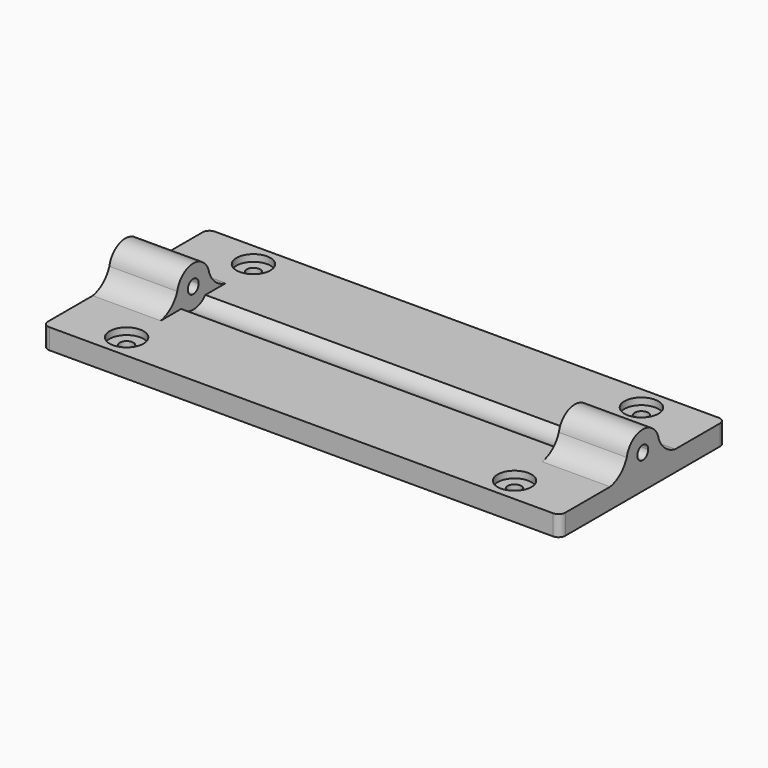
from build123d import *

# Parameters (mm, degrees)
F0_W          = 76.2
F0_H          = 30.48
F0_R          = 2.5
F2_DEPTH      = 3
F0_R_2        = 1
F3_DEPTH      = 2
F4_START      = 28.1
F4_DEPTH      = 10
F5_START      = -28.1
F5_DEPTH      = 10
F6_DEPTH      = 28.1
F6_DEPTH_BACK = 28.1
F7_R          = 1


with BuildPart() as f2:
    # F0 (on Top) → F2 (new body)
    with BuildSketch(Plane.XY):
        with Locations((0, 1.624652555)):
            Rectangle(F0_W, F0_H)
        with Locations((-28.57, -10.055347445)):
            Circle(F0_R, mode=Mode.SUBTRACT)
        with Locations((28.57, -10.055347445)):
            Circle(F0_R, mode=Mode.SUBTRACT)
        with Locations((-28.57, 13.304652555)):
            Circle(F0_R, mode=Mode.SUBTRACT)
        with Locations((28.57, 13.304652555)):
            Circle(F0_R, mode=Mode.SUBTRACT)
    extrude(amount=F2_DEPTH)

    # F0 (on Top) → F3 (join)
    with BuildSketch(Plane.XY):
        with Locations((28.57, 13.304652555)):
            Circle(F0_R)
        with Locations((28.57, 13.304652555)):
            Circle(F0_R_2, mode=Mode.SUBTRACT)
        with Locations((28.57, -10.055347445)):
            Circle(F0_R)
        with Locations((28.57, -10.055347445)):
            Circle(F0_R_2, mode=Mode.SUBTRACT)
        with Locations((-28.57, -10.055347445)):
            Circle(F0_R)
        with Locations((-28.57, -10.055347445)):
            Circle(F0_R_2, mode=Mode.SUBTRACT)
        with Locations((-28.57, 13.304652555)):
            Circle(F0_R)
        with Locations((-28.57, 13.304652555)):
            Circle(F0_R_2, mode=Mode.SUBTRACT)
    extrude(amount=F3_DEPTH)

    # F1 (on Right) → F4 (join)
    with BuildSketch(Plane.YZ.offset(F4_START)):
        with BuildLine():
            ThreePointArc((-1.3122499903, 5.5619300567), (-2.4969921778, 3.8736281168), (-4.365347445, 3))
            Line((-4.365347445, 3), (-0.6014154225, 3))
            ThreePointArc((-0.6014154225, 3), (-1.2561375211, 4.1979197446), (-1.3122499903, 5.5619300567))
        make_face()
        with BuildLine():
            Line((3.8707205325, 3), (7.634652555, 3))
            ThreePointArc((7.634652555, 3), (5.7662972877, 3.8736281168), (4.5815551003, 5.5619300567))
            ThreePointArc((4.5815551003, 5.5619300567), (4.6213486925, 5.2822165518), (4.634652555, 5))
            ThreePointArc((4.634652555, 5), (4.4371696319, 3.9295337307), (3.8707205325, 3))
        make_face()
        with BuildLine():
            ThreePointArc((-1.3122499903, 5.5619300567), (-1.2561375211, 4.1979197446), (-0.6014154225, 3))
            Line((-0.6014154225, 3), (3.8707205325, 3))
            ThreePointArc((3.8707205325, 3), (4.4371696319, 3.9295337307), (4.634652555, 5))
            ThreePointArc((4.634652555, 5), (4.6213486925, 5.2822165518), (4.5815551003, 5.5619300567))
            ThreePointArc((4.5815551003, 5.5619300567), (1.634652555, 8), (-1.3122499903, 5.5619300567))
        make_face()
        with BuildLine():
            ThreePointArc((1.634652555, 4), (0.9275457738, 5.7071067812), (2.634652555, 5))
            ThreePointArc((2.634652555, 5), (2.3417593362, 4.2928932188), (1.634652555, 4))
        make_face(mode=Mode.SUBTRACT)
    extrude(amount=F4_DEPTH)

    # F1 (on Right) → F5 (join)
    with BuildSketch(Plane.YZ.offset(F5_START)):
        with BuildLine():
            ThreePointArc((-1.3122499903, 5.5619300567), (-2.4969921778, 3.8736281168), (-4.365347445, 3))
            Line((-4.365347445, 3), (-0.6014154225, 3))
            ThreePointArc((-0.6014154225, 3), (-1.2561375211, 4.1979197446), (-1.3122499903, 5.5619300567))
        make_face()
        with BuildLine():
            Line((3.8707205325, 3), (7.634652555, 3))
            ThreePointArc((7.634652555, 3), (5.7662972877, 3.8736281168), (4.5815551003, 5.5619300567))
            ThreePointArc((4.5815551003, 5.5619300567), (4.6213486925, 5.2822165518), (4.634652555, 5))
            ThreePointArc((4.634652555, 5), (4.4371696319, 3.9295337307), (3.8707205325, 3))
        make_face()
        with BuildLine():
            ThreePointArc((-1.3122499903, 5.5619300567), (-1.2561375211, 4.1979197446), (-0.6014154225, 3))
            Line((-0.6014154225, 3), (3.8707205325, 3))
            ThreePointArc((3.8707205325, 3), (4.4371696319, 3.9295337307), (4.634652555, 5))
            ThreePointArc((4.634652555, 5), (4.6213486925, 5.2822165518), (4.5815551003, 5.5619300567))
            ThreePointArc((4.5815551003, 5.5619300567), (1.634652555, 8), (-1.3122499903, 5.5619300567))
        make_face()
        with BuildLine():
            ThreePointArc((1.634652555, 4), (0.9275457738, 5.7071067812), (2.634652555, 5))
            ThreePointArc((2.634652555, 5), (2.3417593362, 4.2928932188), (1.634652555, 4))
        make_face(mode=Mode.SUBTRACT)
    extrude(amount=-F5_DEPTH)

    # F1 (on Right) → F6 (cut, two sides)
    with BuildSketch(Plane.YZ) as f6_sk:
        with BuildLine():
            Line((3.8707205325, 3), (-0.6014154225, 3))
            ThreePointArc((-0.6014154225, 3), (1.634652555, 2), (3.8707205325, 3))
        make_face()
    extrude(amount=-F6_DEPTH, mode=Mode.SUBTRACT)
    extrude(f6_sk.sketch, amount=F6_DEPTH_BACK, mode=Mode.SUBTRACT)

    # F7
    f7_edges = [f2.edges().sort_by_distance(p)[0] for p in [
        (38.1, -13.615347, 1.5),
        (38.1, 16.864653, 1.5),
        (-38.1, 16.864653, 1.5),
        (-38.1, -13.615347, 1.5),
    ]]
    fillet(f7_edges, radius=F7_R)


solid = f2.part
